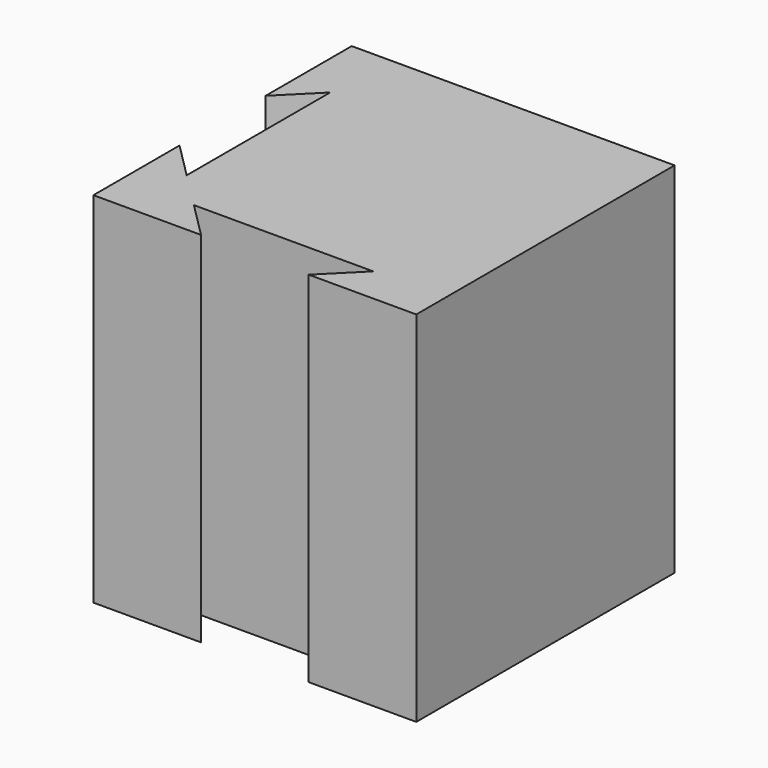
from build123d import *

# Parameters (mm, degrees)
F1_DEPTH = 50


# Not quite as in the source:
# - a feature names something its author has since deleted; it is built from what else it names


with BuildPart() as f1:
    # F0 (on Top) → F1 (new body)
    with BuildSketch(Plane.XY):
        Polygon((-6.1280163284, 19.2819308888), (-21.1280163284, 19.2819308888), (-21.1280163284, 4.2819308888), (-16.1280163284, 9.2819308888), (-16.1280163284, -15.7180691112), (-21.1280163284, -10.7180691112), (-21.1280163284, -25.7180691112), (-6.1280163284, -25.7180691112), (-11.1280163284, -20.7180691112), (13.8719836716, -20.7180691112), (8.8719836716, -25.7180691112), (23.8719836716, -25.7180691112), (23.8719836716, -10.7180691112), (23.8719836716, 4.2819308888), (23.8719836716, 19.2819308888), (8.8719836716, 19.2819308888), align=None)
    extrude(amount=F1_DEPTH)


solid = f1.part
